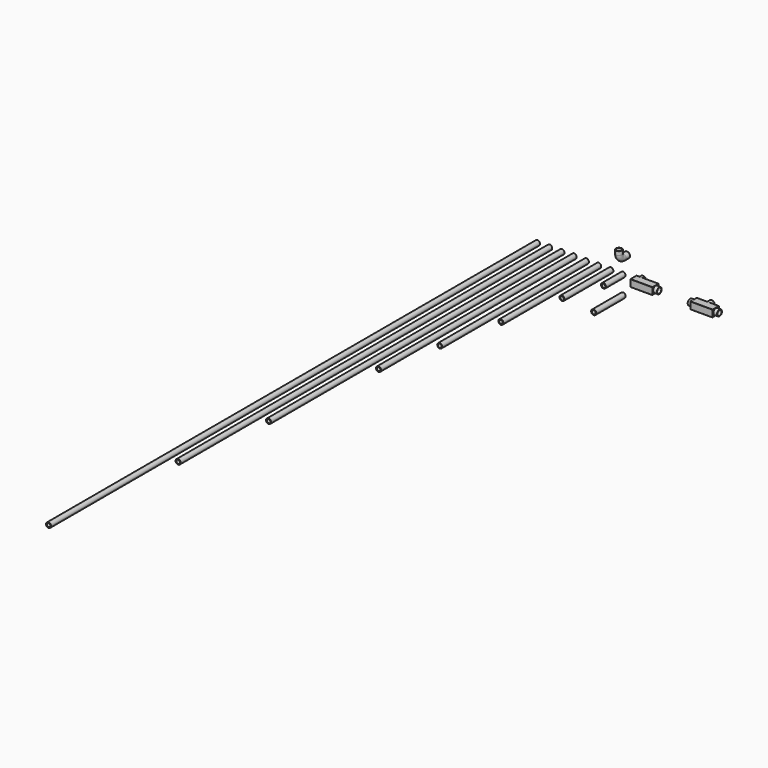
from build123d import *

# Parameters (mm, degrees)
F0_R        = 10.2746162667
F0_R_2      = 7.2636748813
F1_DEPTH    = 100
F2_DEPTH    = 250
F3_DEPTH    = 500
F4_DEPTH    = 750
F5_DEPTH    = 1000
F6_DEPTH    = 1500
F7_DEPTH    = 1900
F8_DEPTH    = 2500
F0_R_3      = 12.25
F0_R_4      = 10.4926415245
F9_DEPTH    = 15
F0_W        = 90
F0_H        = 28
F0_W_2      = 87
F0_H_2      = 24.8196627945
F9_FACE_R   = 12.25
F9_FACE_R_2 = 10.4926415245
F10_DEPTH   = 3
F11_DEPTH   = 30
F12_DEPTH   = 3
F13_W       = 91
F13_H       = 29
F14_DEPTH   = 2
F16_R       = 12.5
F16_R_2     = 10.5
F17_DEPTH   = 15
F18_R       = 1
F0_R_5      = 12.5
F0_R_6      = 10.5
F19_DEPTH   = 20
F0_R_7      = 7.5
F22_DEPTH   = 150
F23_DEPTH   = 20
F24_DEPTH   = 3
F25_DEPTH   = 30
F26_R       = 10.4418172779
F27_DEPTH   = 15
F28_D       = 20.5
F28_DEPTH   = 100
F28_TIP     = 6.158821345
F29_R       = 12.5
F29_R_2     = 10.25
F30_DEPTH   = 15
F31_W       = 91
F31_H       = 29
F31_W_2     = 90
F31_H_2     = 28
F31_W_3     = 87
F31_H_3     = 24.8196627945
F32_DEPTH   = 3
F33_R       = 1


# Not quite as in the source:
# - after a boolean that leaves OpenCascade's solid faulty, fix() repairs it


with BuildPart() as f1:
    # F0 (on Front) → F1 (new body)
    with BuildSketch(Plane.XZ):
        Circle(F0_R)
        Circle(F0_R_2, mode=Mode.SUBTRACT)
    extrude(amount=F1_DEPTH)


with BuildPart() as f2:
    # F0 (on Front) → F2 (new body)
    with BuildSketch(Plane.XZ):
        with Locations((-49.8517975211, -0.1028322222)):
            Circle(F0_R)
        with Locations((-49.8517975211, -0.1028322222)):
            Circle(F0_R_2, mode=Mode.SUBTRACT)
    extrude(amount=F2_DEPTH)


with BuildPart() as f3:
    # F0 (on Front) → F3 (new body)
    with BuildSketch(Plane.XZ):
        with Locations((-99.7955575585, -0.1904692035)):
            Circle(F0_R)
        with Locations((-99.7955575585, -0.1904692035)):
            Circle(F0_R_2, mode=Mode.SUBTRACT)
    extrude(amount=F3_DEPTH)


with BuildPart() as f4:
    # F0 (on Front) → F4 (new body)
    with BuildSketch(Plane.XZ):
        with Locations((-149.9361395836, -0.455326488)):
            Circle(F0_R)
        with Locations((-149.9361395836, -0.455326488)):
            Circle(F0_R_2, mode=Mode.SUBTRACT)
    extrude(amount=F4_DEPTH)


with BuildPart() as f5:
    # F0 (on Front) → F5 (new body)
    with BuildSketch(Plane.XZ):
        with Locations((-200.2543956041, 0.7034467999)):
            Circle(F0_R)
        with Locations((-200.2543956041, 0.7034467999)):
            Circle(F0_R_2, mode=Mode.SUBTRACT)
    extrude(amount=F5_DEPTH)


with BuildPart() as f6:
    # F0 (on Front) → F6 (new body)
    with BuildSketch(Plane.XZ):
        with Locations((-250.1658499241, 0.211708757)):
            Circle(F0_R)
        with Locations((-250.1658499241, 0.211708757)):
            Circle(F0_R_2, mode=Mode.SUBTRACT)
    extrude(amount=F6_DEPTH)


with BuildPart() as f7:
    # F0 (on Front) → F7 (new body)
    with BuildSketch(Plane.XZ):
        with Locations((-300.0773489475, 0.2117086115)):
            Circle(F0_R)
        with Locations((-300.0773489475, 0.2117086115)):
            Circle(F0_R_2, mode=Mode.SUBTRACT)
    extrude(amount=F7_DEPTH)


with BuildPart() as f8:
    # F0 (on Front) → F8 (new body)
    with BuildSketch(Plane.XZ):
        with Locations((-349.9888181686, -0.0341606319)):
            Circle(F0_R)
        with Locations((-349.9888181686, -0.0341606319)):
            Circle(F0_R_2, mode=Mode.SUBTRACT)
    extrude(amount=F8_DEPTH)


with BuildPart() as f9:
    # F0 (on Front) → F9 (new body)
    with BuildSketch(Plane.XZ):
        with Locations((69.7358027101, 0)):
            Circle(F0_R_3)
        with Locations((69.7358027101, 0)):
            Circle(F0_R_4, mode=Mode.SUBTRACT)
    extrude(amount=-F9_DEPTH)

    # F0 (on Front) + F9_face (on face) → F10 (join)
    with BuildSketch(Plane.XZ):
        with Locations((100, 0)):
            Rectangle(F0_W, F0_H)
        with Locations((100, 0)):
            Rectangle(F0_W_2, F0_H_2, mode=Mode.SUBTRACT)
    with BuildSketch(Plane(origin=(69.7358027101, 0, 0), x_dir=(1, 0, 0), z_dir=(0, -1, 0))):
        Circle(F9_FACE_R)
        Circle(F9_FACE_R_2, mode=Mode.SUBTRACT)
    extrude(amount=F10_DEPTH)

    # F0 (on Front) → F11 (join)
    with BuildSketch(Plane.XZ):
        with Locations((100, 0)):
            Rectangle(F0_W, F0_H)
        with Locations((100, 0)):
            Rectangle(F0_W_2, F0_H_2, mode=Mode.SUBTRACT)
    extrude(amount=F11_DEPTH)

    # F0 (on Front) → F12 (join)
    with BuildSketch(Plane.XZ):
        with Locations((100, 0)):
            Rectangle(F0_W_2, F0_H_2)
        with Locations((69.7358027101, 0)):
            Circle(F0_R_3, mode=Mode.SUBTRACT)
        with Locations((69.7358027101, 0)):
            Circle(F0_R_3)
        with Locations((69.7358027101, 0)):
            Circle(F0_R_4, mode=Mode.SUBTRACT)
    extrude(amount=F12_DEPTH)

    # F13 (on face) → F14 (join)
    with BuildSketch(Plane.XZ.offset(30)):
        with Locations((99.9999986887, 4.172e-07)):
            Rectangle(F13_W, F13_H)
    extrude(amount=F14_DEPTH)

    # F16 (on offset) → F17 (join)
    with BuildSketch(Plane.YZ.offset(145)):
        with Locations((-15.1358721778, 0)):
            Circle(F16_R)
        with Locations((-15.1358721778, 0)):
            Circle(F16_R_2, mode=Mode.SUBTRACT)
    extrude(amount=F17_DEPTH)

    # F18
    f18_edges = [f9.edges().sort_by_distance(p)[0] for p in [
        (145.499999, -32, 0),
        (99.999999, -32, 14.5),
        (54.499999, -32, 0),
        (99.999999, -32, -14.5),
    ]]
    fillet(f18_edges, radius=F18_R)


with BuildPart() as f19:
    # F0 (on Front) → F19 (new body)
    with BuildSketch(Plane.XZ):
        with Locations((0, 62.6385882497)):
            Circle(F0_R_5)
        with Locations((0, 62.6385882497)):
            Circle(F0_R_6, mode=Mode.SUBTRACT)
    extrude(amount=-F19_DEPTH)

    # F21: sweep along a path in F20
    with BuildLine(Plane.YZ) as f21_path:
        ThreePointArc((0, 62.6426339149), (-14.8492424049, 68.79339151), (-21, 83.6426339149))
        Line((-21, 83.6426339149), (-21, 98.6426339149))
    # F0 (on Front) → F21 (sweep)
    with BuildSketch(Plane.XZ):
        with Locations((0, 62.6385882497)):
            Circle(F0_R_5)
        with Locations((0, 62.6385882497)):
            Circle(F0_R_6, mode=Mode.SUBTRACT)
    sweep(path=f21_path.line)


with BuildPart() as f22:
    # F0 (on Front) → F22 (new body)
    with BuildSketch(Plane.XZ):
        with Locations((0, -75)):
            Circle(F0_R_6)
        with Locations((0, -75)):
            Circle(F0_R_7, mode=Mode.SUBTRACT)
    extrude(amount=F22_DEPTH)


with BuildPart() as f23:
    # F0 (on Front) → F23 (new body)
    with BuildSketch(Plane.XZ):
        with Locations((346.343113184, 0)):
            Circle(F0_R_3)
        with Locations((346.343113184, 0)):
            Circle(F0_R_4, mode=Mode.SUBTRACT)
    extrude(amount=-F23_DEPTH)

    # F0 (on Front) → F24 (join)
    with BuildSketch(Plane.XZ):
        with Locations((346.343113184, 0)):
            Rectangle(F0_W, F0_H)
        with Locations((346.343113184, 0)):
            Rectangle(F0_W_2, F0_H_2, mode=Mode.SUBTRACT)
        with Locations((346.343113184, 0)):
            Rectangle(F0_W_2, F0_H_2)
        with Locations((346.343113184, 0)):
            Circle(F0_R_3, mode=Mode.SUBTRACT)
        with Locations((346.343113184, 0)):
            Circle(F0_R_3)
        with Locations((346.343113184, 0)):
            Circle(F0_R_4, mode=Mode.SUBTRACT)
    extrude(amount=F24_DEPTH)

    # F0 (on Front) → F25 (join)
    with BuildSketch(Plane.XZ):
        with Locations((346.343113184, 0)):
            Rectangle(F0_W, F0_H)
        with Locations((346.343113184, 0)):
            Rectangle(F0_W_2, F0_H_2, mode=Mode.SUBTRACT)
    extrude(amount=F25_DEPTH)

    # F26 (on face) → F27 (join)
    with BuildSketch(Plane.YZ.offset(391.343113184)):
        with BuildLine():
            ThreePointArc((-3, -3.0864597825), (-2.7106056582, -1.5552739167), (-2.6136402784, 0))
            ThreePointArc((-2.6136402784, 0), (-2.7106056582, 1.5552739167), (-3, 3.0864597825))
            Line((-3, 3.0864597825), (-3, -3.0864597825))
        make_face()
        with BuildLine():
            Line((-3, -3.0864597825), (-3, 3.0864597825))
            ThreePointArc((-3, 3.0864597825), (-27.6563848557, 0), (-3, -3.0864597825))
        make_face()
        with Locations((-15.135012567, 0)):
            Circle(F26_R, mode=Mode.SUBTRACT)
    extrude(amount=F27_DEPTH)

    # F28
    with Locations(Plane.YZ.offset(391.343113184)):
        with Locations((-15.135012567, 0)):
            Hole(F28_D / 2, depth=F28_DEPTH)
            with Locations((0, 0, -(F28_DEPTH + F28_TIP / 2))):  # 118° drill point
                Cone(0, F28_D / 2, F28_TIP, mode=Mode.SUBTRACT)

    # F29 (on face) → F30 (join)
    with BuildSketch(Plane(origin=(301.343113184, 0, 0), x_dir=(0, -1, 0), z_dir=(-1, 0, 0))):
        with Locations((15.135012567, 0)):
            Circle(F29_R)
        with Locations((15.135012567, 0)):
            Circle(F29_R_2, mode=Mode.SUBTRACT)
    extrude(amount=F30_DEPTH)

    # F31 (on face) → F32 (join)
    with BuildSketch(Plane.XZ.offset(30)):
        with Locations((346.343113184, -4.172e-07)):
            Rectangle(F31_W, F31_H)
        with Locations((346.343113184, 0)):
            Rectangle(F31_W_2, F31_H_2, mode=Mode.SUBTRACT)
        with Locations((346.343113184, 0)):
            Rectangle(F31_W_2, F31_H_2)
        with Locations((346.343113184, 0)):
            Rectangle(F31_W_3, F31_H_3, mode=Mode.SUBTRACT)
        with Locations((346.343113184, 0)):
            Rectangle(F31_W_3, F31_H_3)
    extrude(amount=F32_DEPTH)

    add(f23.part.fix(), mode=Mode.REPLACE)

    # F33
    f33_edges = [f23.edges().sort_by_distance(p)[0] for p in [
        (391.843113, -33, 0),
        (346.343113, -33, 14.5),
        (300.843113, -33, 0),
        (346.343113, -33, -14.5),
    ]]
    fillet(f33_edges, radius=F33_R)


solid = Compound([f1.part, f2.part, f3.part, f4.part, f5.part, f6.part, f7.part, f8.part, f9.part, f19.part, f22.part, f23.part])
